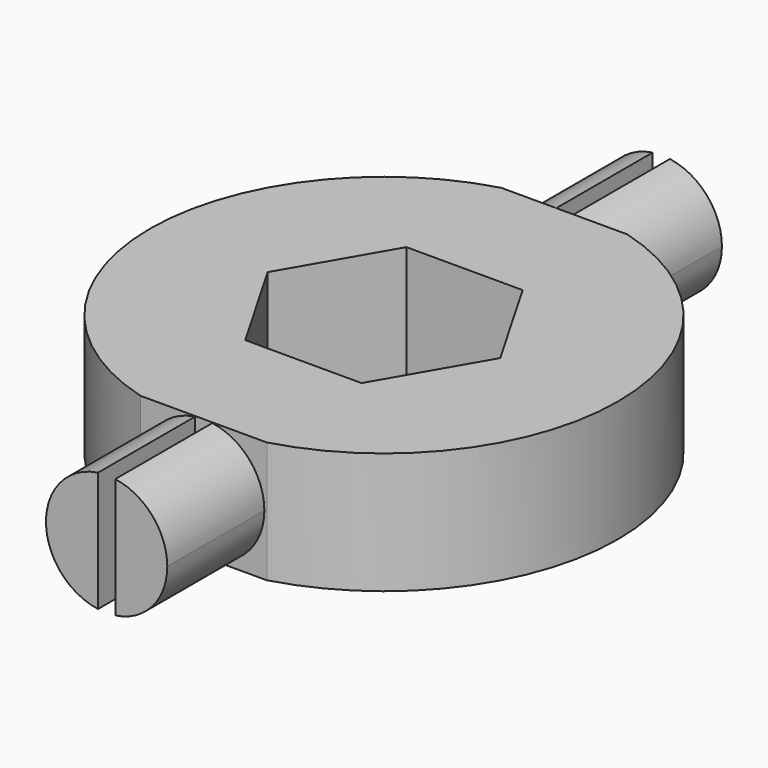
from build123d import *

# Parameters (mm, degrees)
F1_DEPTH = 7
F3_DEPTH = 7


# Not quite as in the source:
# - a pattern or mirror of a feature is missing from the dataset's text; its kind, count and spacing are read off the source's solid


with BuildPart() as f1:
    # F0 (on Top) → F1 (new body)
    with BuildSketch(Plane.XY):
        with BuildLine():
            Line((3.6400549446, 13), (-3.6400549446, 13))
            ThreePointArc((-3.6400549446, 13), (-13.5, 0), (-3.6400549446, -13))
            Line((-3.6400549446, -13), (3.6400549446, -13))
            ThreePointArc((3.6400549446, -13), (13.5, 0), (3.6400549446, 13))
        make_face()
        Polygon((-6.7091866291, 0), (-3.3545933146, 5.8103260596), (3.3545933146, 5.8103260596), (6.7091866291, 0), (3.3545933146, -5.8103260596), (-3.3545933146, -5.8103260596), align=None, mode=Mode.SUBTRACT)
    extrude(amount=F1_DEPTH)

    # F2 (on face) → F3 (join)
    with BuildSketch(Plane.XZ.offset(13)):
        with BuildLine():
            Line((-0.5, 0.0358983849), (-0.5, 6.9641016151))
            ThreePointArc((-0.5, 6.9641016151), (-3.5, 3.5), (-0.5, 0.0358983849))
        make_face()
        with BuildLine():
            ThreePointArc((0.5, 0.0358983849), (2.6457513111, 1.2087121525), (3.5, 3.5))
            ThreePointArc((3.5, 3.5), (2.6457513111, 5.7912878475), (0.5, 6.9641016151))
            Line((0.5, 6.9641016151), (0.5, 0.0358983849))
        make_face()
    f3 = extrude(amount=F3_DEPTH)

    # F3_copies: F3 across plane
    add(f3.mirror(Plane.ZX))


solid = f1.part
